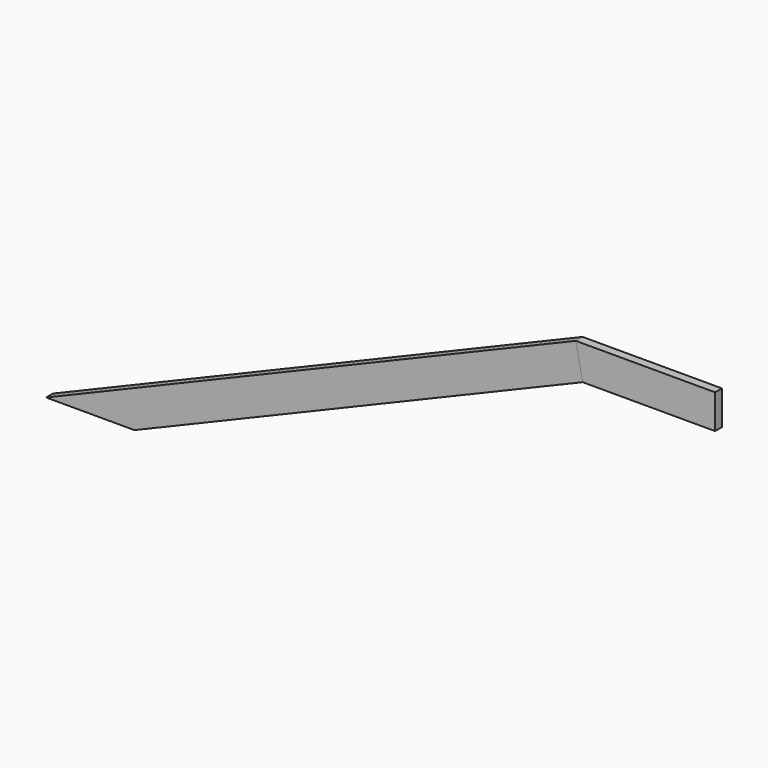
from build123d import *

# Parameters (mm, degrees)
F1_DEPTH = 25.4
F2_DEPTH = 25.4


# Not quite as in the source:
# - a feature names something its author has since deleted; it is built from what else it names


with BuildPart() as f1:
    # F0 (on Front) → F1 (new body)
    with BuildSketch(Plane.XZ):
        Polygon((1574.8, 660.4), (0, 0), (262.7178476153, 0), (1574.8, 550.2279993871), align=None)
        Polygon((1595.2409245384, 558.8), (1574.8, 660.4), (1574.8, 550.2279993871), align=None)
    extrude(amount=F1_DEPTH)


with BuildPart() as f2:
    # F0 (on Front) → F2 (new body)
    with BuildSketch(Plane.XZ):
        Polygon((1988.9409245384, 660.4), (1574.8, 660.4), (1595.2409245384, 558.8), (1988.9409245384, 558.8), align=None)
    extrude(amount=F2_DEPTH)


solid = Compound([f1.part, f2.part])
